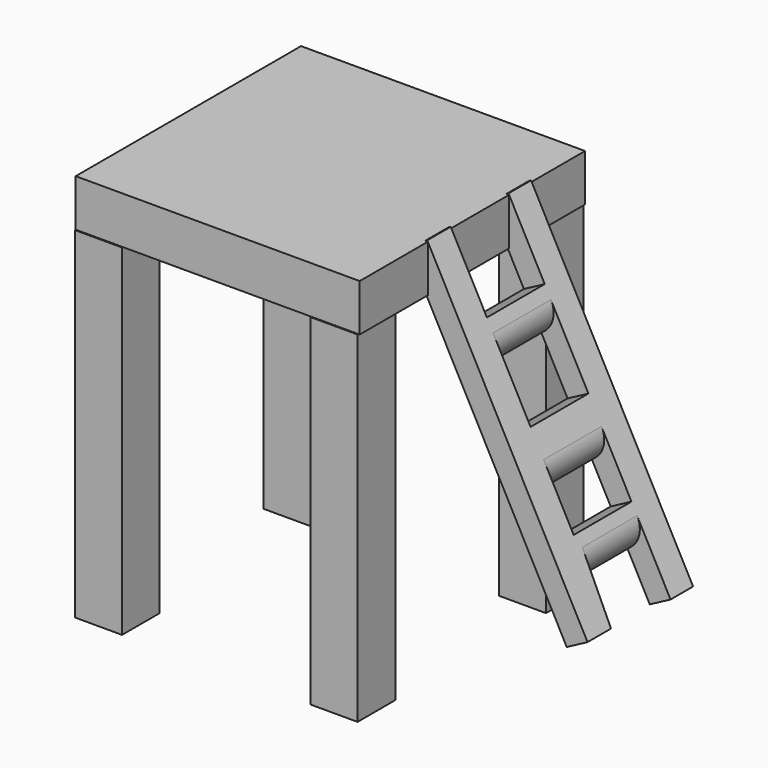
from build123d import *

# Parameters (mm, degrees)
F0_W     = 10
F0_H     = 10
F1_DEPTH = 72.4
F2_W     = 60.2884615958
F2_H     = 59.7972988337
F3_DEPTH = 10
F5_W     = 15.3336008079
F5_H     = 8.5764247924
F5_H_2   = 11.9550051168
F6_DEPTH = 5
F7_R     = 4.99999


# Not quite as in the source:
# - a fillet or chamfer is up to 0.001 mm smaller than in the source, because OpenCascade refuses the exact size


with BuildPart() as f1:
    # F0 (on Top) → F1 (new body)
    with BuildSketch(Plane.XY):
        with Locations((25, 25)):
            Rectangle(F0_W, F0_H)
    extrude(amount=F1_DEPTH)


with BuildPart() as f1b:
    # F0 (on Top) → F1, piece 2 (new body)
    with BuildSketch(Plane.XY):
        with Locations((-25, 25)):
            Rectangle(F0_W, F0_H)
    extrude(amount=F1_DEPTH)


with BuildPart() as f1c:
    # F0 (on Top) → F1, piece 3 (new body)
    with BuildSketch(Plane.XY):
        with Locations((25, -25)):
            Rectangle(F0_W, F0_H)
    extrude(amount=F1_DEPTH)


with BuildPart() as f1d:
    # F0 (on Top) → F1, piece 4 (new body)
    with BuildSketch(Plane.XY):
        with Locations((-25, -25)):
            Rectangle(F0_W, F0_H)
    extrude(amount=F1_DEPTH)


with BuildPart() as f3:
    # F2 (on face) → F3 (new body)
    with BuildSketch(Plane.XY.offset(72.4)):
        with Locations((0.1442307979, 0.1013505831)):
            Rectangle(F2_W, F2_H)
    extrude(amount=F3_DEPTH)

    # F5 (on face) → F6 (join)
    with BuildSketch(Plane(origin=(57.7655486917, 0, 30.7018579048), x_dir=(0, 1, 0), z_dir=(0.8830276047, 0, 0.4693210514))):
        Polygon((-5.4863165133, 58.8063634932), (-11.7237139493, 58.8063634932), (-11.7237139493, -13.7033779174), (-5.4863165133, -13.7033779174), (-4.9665332772, -4.3472838588), (9.8472842947, -4.3472838588), (9.8472842947, -14.4830560312), (15.824791044, -14.4830560312), (15.824791044, 58.8063634932), (9.8472842947, 58.8063634932), (9.8472842947, 42.4331985414), (-5.4863165133, 42.4331985414), align=None)
        with Locations((2.1804838907, 7.4777789414)):
            Rectangle(F5_W, F5_H, mode=Mode.SUBTRACT)
        with Locations((2.1804838907, 28.6589427851)):
            Rectangle(F5_W, F5_H_2, mode=Mode.SUBTRACT)
    extrude(amount=-F6_DEPTH)

    # F7 (radius 5 in the source; OpenCascade refuses exactly that, so slightly less here)
    f7_edges = [f3.edges().sort_by_distance(p)[0] for p in [
        (41.509936, 2.180484, 61.286795),
        (52.243521, 2.180484, 41.091553),
        (59.805821, 2.440376, 26.863086),
    ]]
    fillet(f7_edges, radius=F7_R)


solid = Compound([f1.part, f1b.part, f1c.part, f1d.part, f3.part])
